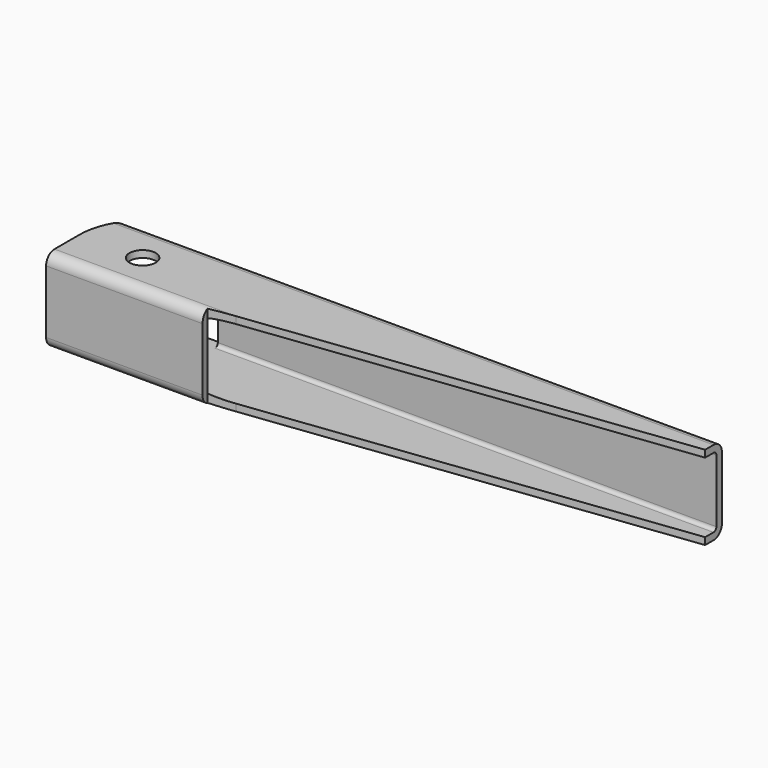
from build123d import *

# Parameters (mm, degrees)
F1_DEPTH = 184.15
F3_DEPTH = 33.3375
F4_R     = 3.96875
F5_DEPTH = 25.401
F7_DEPTH = 25.401
F9_DEPTH = 25.4010001


with BuildPart() as f1:
    # F0 (on Right) → F1 (new body)
    with BuildSketch(Plane.YZ):
        with BuildLine():
            Line((-9.525, -12.7), (9.525, -12.7))
            ThreePointArc((9.525, -12.7), (11.7700640303, -11.7700640303), (12.7, -9.525))
            Line((12.7, -9.525), (12.7, 9.525))
            ThreePointArc((12.7, 9.525), (11.7700640303, 11.7700640303), (9.525, 12.7))
            Line((9.525, 12.7), (-9.525, 12.7))
            ThreePointArc((-9.525, 12.7), (-11.7700640303, 11.7700640303), (-12.7, 9.525))
            Line((-12.7, 9.525), (-12.7, -9.525))
            ThreePointArc((-12.7, -9.525), (-11.7700640303, -11.7700640303), (-9.525, -12.7))
        make_face()
        with BuildLine():
            Line((-9.525, 10.5918), (9.525, 10.5918))
            ThreePointArc((9.525, 10.5918), (10.2793415142, 10.2793415142), (10.5918, 9.525))
            Line((10.5918, 9.525), (10.5918, -9.525))
            ThreePointArc((10.5918, -9.525), (10.2793415142, -10.2793415142), (9.525, -10.5918))
            Line((9.525, -10.5918), (-9.525, -10.5918))
            ThreePointArc((-9.525, -10.5918), (-10.2793415142, -10.2793415142), (-10.5918, -9.525))
            Line((-10.5918, -9.525), (-10.5918, 9.525))
            ThreePointArc((-10.5918, 9.525), (-10.2793415142, 10.2793415142), (-9.525, 10.5918))
        make_face(mode=Mode.SUBTRACT)
    extrude(amount=F1_DEPTH)

    # F2 (on face) → F3 (cut)
    with BuildSketch(Plane(origin=(0, 0, 0), x_dir=(0, -1, 0), z_dir=(-1, 0, 0))):
        with BuildLine():
            ThreePointArc((-12.7, 9.525), (-12.6535126242, 10.0663259281), (-12.5154118044, 10.5918))
            Line((-12.5154118044, 10.5918), (-16.0259325057, 10.5918))
            Line((-16.0259325057, 10.5918), (-16.0259325057, -10.5918))
            Line((-16.0259325057, -10.5918), (-12.5154118044, -10.5918))
            ThreePointArc((-12.5154118044, -10.5918), (-12.6535126242, -10.0663259281), (-12.7, -9.525))
            Line((-12.7, -9.525), (-12.7, 9.525))
        make_face()
        with BuildLine():
            Line((-7.5196851976, -10.5918), (-7.5196851976, 10.5918))
            Line((-7.5196851976, 10.5918), (-9.525, 10.5918))
            ThreePointArc((-9.525, 10.5918), (-10.2793415142, 10.2793415142), (-10.5918, 9.525))
            Line((-10.5918, 9.525), (-10.5918, -9.525))
            ThreePointArc((-10.5918, -9.525), (-10.2793415142, -10.2793415142), (-9.525, -10.5918))
            Line((-9.525, -10.5918), (-7.5196851976, -10.5918))
        make_face()
        with BuildLine():
            ThreePointArc((-10.5918, 9.525), (-10.2793415142, 10.2793415142), (-9.525, 10.5918))
            Line((-9.525, 10.5918), (-12.5154118044, 10.5918))
            ThreePointArc((-12.5154118044, 10.5918), (-12.6535126242, 10.0663259281), (-12.7, 9.525))
            Line((-12.7, 9.525), (-12.7, -9.525))
            ThreePointArc((-12.7, -9.525), (-12.6535126242, -10.0663259281), (-12.5154118044, -10.5918))
            Line((-12.5154118044, -10.5918), (-9.525, -10.5918))
            ThreePointArc((-9.525, -10.5918), (-10.2793415142, -10.2793415142), (-10.5918, -9.525))
            Line((-10.5918, -9.525), (-10.5918, 9.525))
        make_face()
    extrude(amount=-F3_DEPTH, mode=Mode.SUBTRACT)

    # F4 (on face) → F5 (cut, through all)
    with BuildSketch(Plane.XY.offset(12.7)):
        with Locations((19.05, 0)):
            Circle(F4_R)
    extrude(amount=-F5_DEPTH, mode=Mode.SUBTRACT)

    # F6 (on face) → F7 (cut, through all)
    with BuildSketch(Plane.XY.offset(12.7)):
        with BuildLine():
            ThreePointArc((2.5522160579, 9.525), (4.2134911079, 11.9490796254), (6.2278308065, 14.0888068044))
            Line((6.2278308065, 14.0888068044), (1.4018084571, 20.3806743289))
            ThreePointArc((1.4018084571, 20.3806743289), (-5.47164532, 11.203546833), (-7.9097950815, 0))
            Line((-7.9097950815, 0), (0, 0))
            Line((0, 0), (0, 9.525))
            Line((0, 9.525), (2.5522160579, 9.525))
        make_face()
        with BuildLine():
            ThreePointArc((0, 0), (0.6491130092, 4.9305028092), (2.5522160579, 9.525))
            Line((2.5522160579, 9.525), (0, 9.525))
            Line((0, 9.525), (0, 0))
        make_face()
    extrude(amount=-F7_DEPTH, mode=Mode.SUBTRACT)

    # F8 (on face) → F9 (cut, through all)
    with BuildSketch(Plane.XY.offset(12.7)):
        Polygon((184.15, -9.525), (184.15, 6.35), (54.8585004559, -9.525), align=None)
        Polygon((188.5616199521, -29.5797611986), (184.15, 6.35), (184.15, -9.525), (54.8585004559, -9.525), (47.0669696314, -10.481679691), (51.4785895836, -46.4114408897), align=None)
    extrude(amount=-F9_DEPTH, mode=Mode.SUBTRACT)


solid = f1.part
